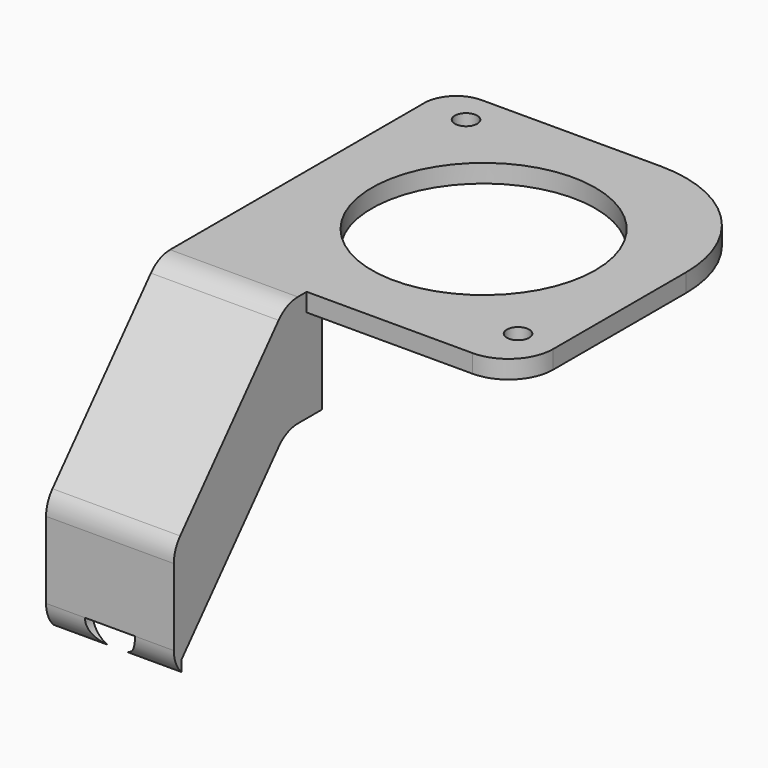
from build123d import *

# Parameters (mm, degrees)
F0_R         = 1.75
F0_R_2       = 17.5
F1_DEPTH     = 2.85
F2_W         = 20
F2_H         = 4
F3_DEPTH     = 14.6
F4_W         = 17
F4_H         = 12.41
F5_DEPTH     = 25
F3_FACE1_W   = 20
F3_FACE1_H   = 17.45
F3_FACE1_W_2 = 17
F3_FACE1_H_2 = 12.41
F9_W         = 20
F9_H         = 17.45
F10_DEPTH    = 1.5
F11_W        = 16.7262982869
F11_H        = 2.3696432114
F12_DEPTH    = 16.4
F13_T1_DEPTH = 20
F13_T3_DEPTH = 31.3016516107
F13_T5_DEPTH = 29.4336950122
F13_T7_DEPTH = 37.8535710714
F4_W_2       = 20
F4_H_2       = 14.6
F14_DEPTH    = 3
F16_DEPTH    = 25


# Not quite as in the source:
# - a fillet or chamfer that OpenCascade refuses, or shapes differently, is made with other operations: its cross-section is extruded or revolved along the edge and cut away or added


with BuildPart() as f1:
    # F0 (on Top) → F1 (new body)
    with BuildSketch(Plane.XY):
        with BuildLine():
            Line((-6.5, -26.5), (19.5, -26.5))
            ThreePointArc((19.5, -26.5), (24.4497474683, -24.4497474683), (26.5, -19.5))
            Line((26.5, -19.5), (26.5, 6.5))
            ThreePointArc((26.5, 6.5), (20.6421356237, 20.6421356237), (6.5, 26.5))
            Line((6.5, 26.5), (-21.5, 26.5))
            ThreePointArc((-21.5, 26.5), (-25.0355339059, 25.0355339059), (-26.5, 21.5))
            Line((-26.5, 21.5), (-26.5, -26.5))
            Line((-26.5, -26.5), (-26.5, -30.5))
            Line((-26.5, -30.5), (-6.5, -30.5))
            Line((-6.5, -30.5), (-6.5, -26.5))
        make_face()
        with Locations((20.6, -19.0101229506)):
            Circle(F0_R, mode=Mode.SUBTRACT)
        with Locations((-19.75, 21.25)):
            Circle(F0_R, mode=Mode.SUBTRACT)
        Circle(F0_R_2, mode=Mode.SUBTRACT)
    extrude(amount=F1_DEPTH)

    # F2 (on face) → F3 (join)
    with BuildSketch(Plane(origin=(0, 0, 0), x_dir=(1, 0, 0), z_dir=(0, 0, -1))):
        with Locations((-16.5, 28.5)):
            Rectangle(F2_W, F2_H)
    extrude(amount=F3_DEPTH)

    # F4 (on face) → F5 (cut)
    with BuildSketch(Plane(origin=(0, -26.5, 0), x_dir=(-1, 0, 0), z_dir=(0, 1, 0))):
        with Locations((16.5, -7.3)):
            Rectangle(F4_W, F4_H)
    extrude(amount=-F5_DEPTH, mode=Mode.SUBTRACT)

    # F8: sweep along a path in F7
    with BuildLine(Plane.YZ.offset(-16.5)) as f8_path:
        Line((-30.5838297752, -0.1396118733), (-52.5838297752, -25.1396118733))
    # F3_face1 (on face) → F8 (sweep)
    with BuildSketch(Plane(origin=(-16.5, -30.5, -3.6969789176), x_dir=(1, 0, 0), z_dir=(0, -1, 0))):
        with Locations((0, -2.1780210824)):
            Rectangle(F3_FACE1_W, F3_FACE1_H)
        with Locations((0, -3.6030210824)):
            Rectangle(F3_FACE1_W_2, F3_FACE1_H_2, mode=Mode.SUBTRACT)
    sweep(path=f8_path.line)

    # F9 (on face) → F10 (join)
    with BuildSketch(Plane.XZ.offset(52.5)):
        with Locations((-16.5, -30.875)):
            Rectangle(F9_W, F9_H)
    extrude(amount=-F10_DEPTH)

    # F11 (on face) → F12 (cut)
    with BuildSketch(Plane(origin=(0, 0, -39.6), x_dir=(1, 0, 0), z_dir=(0, 0, -1))):
        with Locations((-16.5000008565, 49.8151783943)):
            Rectangle(F11_W, F11_H)
    extrude(amount=-F12_DEPTH, mode=Mode.SUBTRACT)

    # F13: fillet of radius 5 on 4 edges, made by hand

    # F13_s2 → F13_t1 (join)
    with BuildSketch(Plane.YZ.offset(-26.5)):
        with BuildLine():
            ThreePointArc((-31.9932372625, -16.2968605255), (-30.299318025, -15.0439217867), (-28.2396696779, -14.6))
            Line((-28.2396696779, -14.6), (-30.5, -14.6))
            Line((-30.5, -14.6), (-31.9932372625, -16.2968605255))
        make_face()
    extrude(amount=F13_T1_DEPTH)

    # F13_s4 → F13_t3 (cut)
    with BuildSketch(Plane.YZ.offset(-32.1508258053)):
        with BuildLine():
            ThreePointArc((-28.2396696779, 2.85), (-30.299318025, 2.4060782133), (-31.9932372625, 1.1531394745))
            Line((-31.9932372625, 1.1531394745), (-30.5, 2.85))
            Line((-30.5, 2.85), (-28.2396696779, 2.85))
        make_face()
    extrude(amount=F13_T3_DEPTH, mode=Mode.SUBTRACT)

    # F13_s6 → F13_t5 (cut)
    with BuildSketch(Plane.YZ.offset(-31.2168475061)):
        with BuildLine():
            ThreePointArc((-52.5, -24.0367390024), (-52.1780251134, -22.2714965153), (-51.2535675846, -20.733599528))
            Line((-51.2535675846, -20.733599528), (-52.5, -22.15))
            Line((-52.5, -22.15), (-52.5, -24.0367390024))
        make_face()
    extrude(amount=F13_T5_DEPTH, mode=Mode.SUBTRACT)

    # F13_s8 → F13_t7 (cut)
    with BuildSketch(Plane.YZ.offset(-35.4267855357)):
        with BuildLine():
            ThreePointArc((-51, -39.6), (-52.1097722286, -37.9657774588), (-52.5, -36.0292857857))
            Line((-52.5, -36.0292857857), (-52.5, -39.6))
            Line((-52.5, -39.6), (-51, -39.6))
        make_face()
    extrude(amount=F13_T7_DEPTH, mode=Mode.SUBTRACT)

    # F4 (on face) → F14 (join)
    with BuildSketch(Plane(origin=(0, -26.5, 0), x_dir=(-1, 0, 0), z_dir=(0, 1, 0))):
        with Locations((16.5, -7.3)):
            Rectangle(F4_W_2, F4_H_2)
        with Locations((16.5, -7.3)):
            Rectangle(F4_W, F4_H, mode=Mode.SUBTRACT)
    extrude(amount=F14_DEPTH)

    # F15 (on face) → F16 (cut)
    with BuildSketch(Plane.XZ.offset(52.5)):
        with BuildLine():
            Line((-12.5835244641, -36.0292857857), (-20.4164755359, -36.0292857857))
            ThreePointArc((-20.4164755359, -36.0292857857), (-16.5, -39.9457613216), (-12.5835244641, -36.0292857857))
        make_face()
    extrude(amount=-F16_DEPTH, mode=Mode.SUBTRACT)


solid = f1.part
